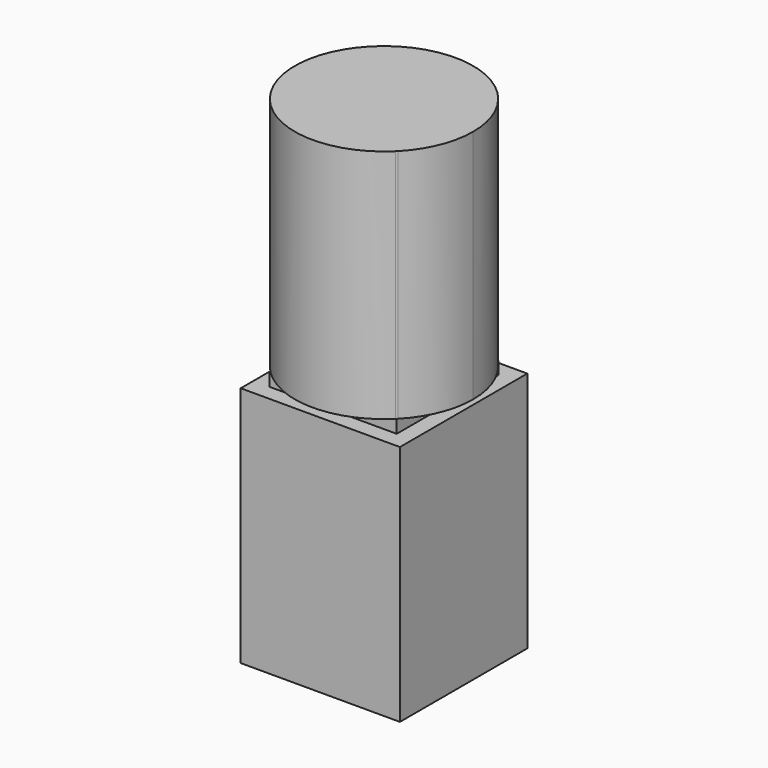
from build123d import *

# Parameters (mm, degrees)
F0_W     = 25
F0_H     = 25
F1_DEPTH = 38
F2_W     = 20
F2_H     = 20
F3_DEPTH = 2
F5_DEPTH = 37


with BuildPart() as f1:
    # F0 (on Top) → F1 (new body)
    with BuildSketch(Plane.XY):
        with Locations((12.5, 12.5)):
            Rectangle(F0_W, F0_H)
    extrude(amount=F1_DEPTH)

    # F2 (on face) → F3 (join)
    with BuildSketch(Plane.XY.offset(38)):
        with Locations((12.5, 12.5)):
            Rectangle(F2_W, F2_H)
    extrude(amount=F3_DEPTH)

    # F4 (on face) → F5 (join)
    with BuildSketch(Plane.XY.offset(40)):
        with BuildLine():
            ThreePointArc((22.5, 2.7020410289), (25.4614813968, 7.2084973779), (26.5, 12.5))
            ThreePointArc((26.5, 12.5), (25.4614813968, 17.7915026221), (22.5, 22.2979589711))
            Line((22.5, 22.2979589711), (22.5, 2.7020410289))
        make_face()
        with BuildLine():
            Line((22.5, 2.7020410289), (22.5, 22.2979589711))
            ThreePointArc((22.5, 22.2979589711), (22.3994949366, 22.3994949366), (22.2979589711, 22.5))
            Line((22.2979589711, 22.5), (2.7020410289, 22.5))
            ThreePointArc((2.7020410289, 22.5), (2.6005050634, 22.3994949366), (2.5, 22.2979589711))
            Line((2.5, 22.2979589711), (2.5, 2.7020410289))
            ThreePointArc((2.5, 2.7020410289), (2.6005050634, 2.6005050634), (2.7020410289, 2.5))
            Line((2.7020410289, 2.5), (22.2979589711, 2.5))
            ThreePointArc((22.2979589711, 2.5), (22.3994949366, 2.6005050634), (22.5, 2.7020410289))
        make_face()
        with BuildLine():
            Line((2.7020410289, 22.5), (22.2979589711, 22.5))
            ThreePointArc((22.2979589711, 22.5), (12.5, 26.5), (2.7020410289, 22.5))
        make_face()
        with BuildLine():
            ThreePointArc((2.7020410289, 2.5), (12.5, -1.5), (22.2979589711, 2.5))
            Line((22.2979589711, 2.5), (2.7020410289, 2.5))
        make_face()
        with BuildLine():
            Line((2.5, 2.7020410289), (2.5, 22.2979589711))
            ThreePointArc((2.5, 22.2979589711), (-1.5, 12.5), (2.5, 2.7020410289))
        make_face()
    extrude(amount=F5_DEPTH)


solid = f1.part
